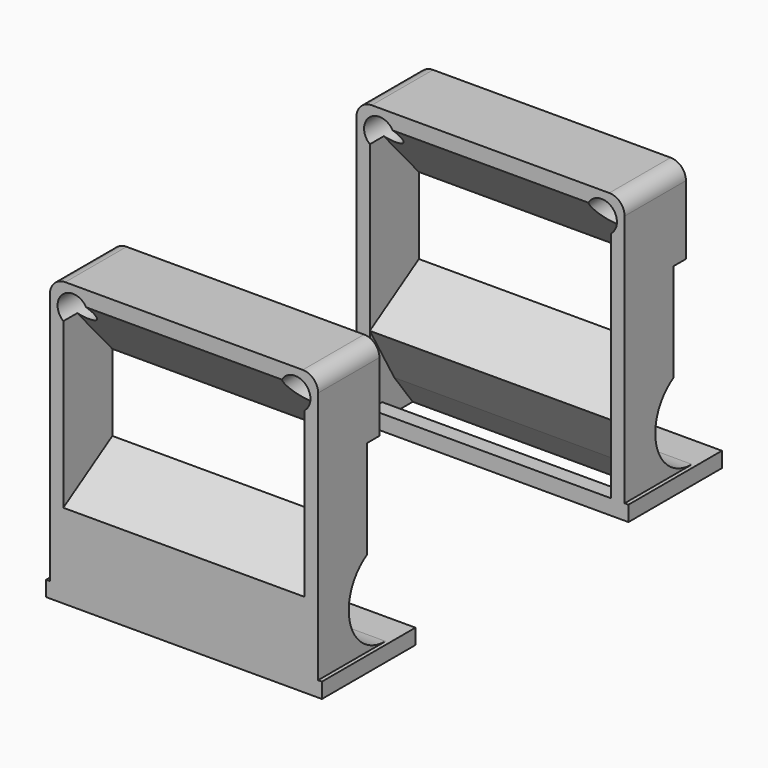
from build123d import *

# Parameters (mm, degrees)
F1_DEPTH      = 35
F2_R          = 2
F3_DEPTH      = 10
F4_R          = 2
F7_DEPTH      = 15.75
F7_DEPTH_BACK = 15.75
F8_W          = 36
F8_H          = 15.25
F8_W_2        = 31.5
F8_H_2        = 5
F9_DEPTH      = 2
F12_DEPTH     = 31.5


with BuildPart() as f1:
    # F0 (on Right) → F1 (new body)
    with BuildSketch(Plane.YZ):
        with BuildLine():
            Line((0, 37), (0, 0))
            Line((0, 0), (15.25, 0))
            Line((15.25, 0), (15.25, 2))
            Line((15.25, 2), (11, 2))
            ThreePointArc((11, 2), (5.2044450423, 6.4470857294), (8, 13.1961524227))
            Line((8, 13.1961524227), (8, 26))
            Line((8, 26), (10, 26))
            Line((10, 26), (10, 37))
            Line((10, 37), (0, 37))
        make_face()
    extrude(amount=F1_DEPTH)

    # F2 (on face) → F3 (cut, through all)
    with BuildSketch(Plane(origin=(0, 10, 0), x_dir=(-1, 0, 0), z_dir=(0, 1, 0))):
        with Locations((-32, 34)):
            Circle(F2_R)
        with Locations((-3, 34)):
            Circle(F2_R)
    extrude(amount=-F3_DEPTH, mode=Mode.SUBTRACT)

    # F4
    f4_edges = [f1.edges().sort_by_distance(p)[0] for p in [
        (0, 5, 37),
        (35, 5, 37),
    ]]
    fillet(f4_edges, radius=F4_R)

    # F6 (on offset) → F7 (cut, two sides)
    with BuildSketch(Plane.YZ.offset(17.5)) as f7_sk:
        Polygon((4, 4), (0, 11), (0, 2), (2, 2), (2, 0), (7, 0), align=None)
        Polygon((8, 26), (0, 35), (0, 11), (8, 16), align=None)
    extrude(amount=F7_DEPTH, mode=Mode.SUBTRACT)
    extrude(f7_sk.sketch, amount=-F7_DEPTH_BACK, mode=Mode.SUBTRACT)

    # F8 (on face) → F9 (join)
    with BuildSketch(Plane(origin=(0, 0, 0), x_dir=(1, 0, 0), z_dir=(0, 0, -1))):
        with Locations((17.5, -7.625)):
            Rectangle(F8_W, F8_H)
        with Locations((17.5, -4.5)):
            Rectangle(F8_W_2, F8_H_2, mode=Mode.SUBTRACT)
    extrude(amount=-F9_DEPTH)


with BuildPart() as f10_1:
    # F10: copy of F1
    add(f1.part.moved(Location((0, -50, 0))))

    # F11 (on face) → F12 (join, through all)
    with BuildSketch(Plane(origin=(33.25, 0, 0), x_dir=(0, -1, 0), z_dir=(-1, 0, 0))):
        Polygon((50, 11), (46, 4), (43, 0), (48, 0), (48, 2), (50, 2), align=None)
    extrude(amount=F12_DEPTH)


solid = Compound([f1.part, f10_1.part])
